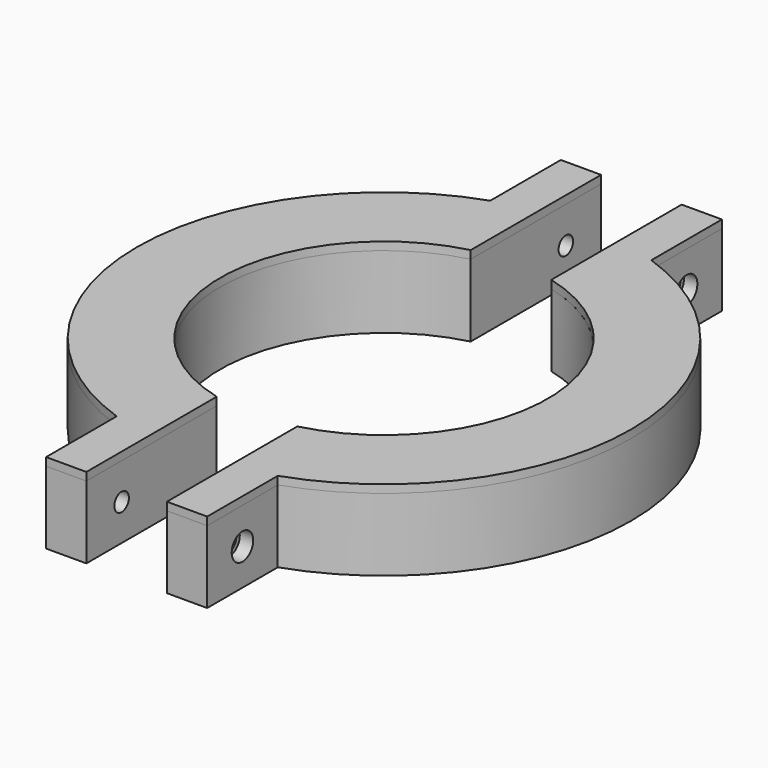
from build123d import *

# Parameters (mm, degrees)
F1_DEPTH      = 2
F2_DEPTH      = 25
F2_DEPTH_BACK = 2
F4_R          = 3.38
F5_DEPTH      = 122.001
F7_DEPTH      = 5
F9_DEPTH      = 3
F6_R          = 5
F6_R_2        = 3.38
F10_DEPTH     = 5


with BuildPart() as f1:
    # F0 (on Top) → F1 (new body)
    with BuildSketch(Plane.XY):
        with BuildLine():
            ThreePointArc((-30, -56.5331761004), (-64, 0), (-30, 56.5331761004))
            Line((-30, 56.5331761004), (-30, 83.7914076741))
            ThreePointArc((-30, 83.7914076741), (-89, 0), (-30, -83.7914076741))
            Line((-30, -83.7914076741), (-30, -56.5331761004))
        make_face()
    extrude(amount=-F1_DEPTH)

    # F0 (on Top) → F2 (join, two sides)
    with BuildSketch(Plane.XY) as f2_sk:
        with BuildLine():
            ThreePointArc((-30, -53.1130868996), (-61, 0), (-30, 53.1130868996))
            Line((-30, 53.1130868996), (-30, 56.5331761004))
            ThreePointArc((-30, 56.5331761004), (-64, 0), (-30, -56.5331761004))
            Line((-30, -56.5331761004), (-30, -53.1130868996))
        make_face()
        with BuildLine():
            ThreePointArc((-30, 53.1130868996), (-22.7000381841, 56.6189744383), (-15, 59.1269819964))
            Line((-15, 59.1269819964), (-15, 62.2173609212))
            ThreePointArc((-15, 62.2173609212), (-22.6787894137, 59.8470760416), (-30, 56.5331761004))
            Line((-30, 56.5331761004), (-30, 53.1130868996))
        make_face()
        with BuildLine():
            Line((-15, -87.7268487978), (-15, -62.2173609212))
            ThreePointArc((-15, -62.2173609212), (-22.6787894137, -59.8470760416), (-30, -56.5331761004))
            Line((-30, -56.5331761004), (-30, -83.7914076741))
            ThreePointArc((-30, -83.7914076741), (-22.5858788673, -86.0864569824), (-15, -87.7268487978))
        make_face()
        with BuildLine():
            Line((-15, -62.2173609212), (-15, -59.1269819964))
            ThreePointArc((-15, -59.1269819964), (-22.7000381841, -56.6189744383), (-30, -53.1130868996))
            Line((-30, -53.1130868996), (-30, -56.5331761004))
            ThreePointArc((-30, -56.5331761004), (-22.6787894137, -59.8470760416), (-15, -62.2173609212))
        make_face()
        with BuildLine():
            Line((-15, -90.768937418), (-15, -87.7268487978))
            ThreePointArc((-15, -87.7268487978), (-22.5858788673, -86.0864569824), (-30, -83.7914076741))
            Line((-30, -83.7914076741), (-30, -86.9712596206))
            ThreePointArc((-30, -86.9712596206), (-22.5799820452, -89.1860101744), (-15, -90.768937418))
        make_face()
        with BuildLine():
            Line((-15, -119.826041162), (-15, -90.768937418))
            ThreePointArc((-15, -90.768937418), (-22.5799820452, -89.1860101744), (-30, -86.9712596206))
            Line((-30, -86.9712596206), (-30, -119.826041162))
            Line((-30, -119.826041162), (-15, -119.826041162))
        make_face()
        with BuildLine():
            ThreePointArc((-30, -83.7914076741), (-89, 0), (-30, 83.7914076741))
            Line((-30, 83.7914076741), (-30, 86.9712596206))
            ThreePointArc((-30, 86.9712596206), (-92, 0), (-30, -86.9712596206))
            Line((-30, -86.9712596206), (-30, -83.7914076741))
        make_face()
        with BuildLine():
            ThreePointArc((-30, 56.5331761004), (-22.6787894137, 59.8470760416), (-15, 62.2173609212))
            Line((-15, 62.2173609212), (-15, 87.7268487978))
            ThreePointArc((-15, 87.7268487978), (-22.5858788673, 86.0864569824), (-30, 83.7914076741))
            Line((-30, 83.7914076741), (-30, 56.5331761004))
        make_face()
        with BuildLine():
            ThreePointArc((-30, 83.7914076741), (-22.5858788673, 86.0864569824), (-15, 87.7268487978))
            Line((-15, 87.7268487978), (-15, 90.768937418))
            ThreePointArc((-15, 90.768937418), (-22.5799820452, 89.1860101744), (-30, 86.9712596206))
            Line((-30, 86.9712596206), (-30, 83.7914076741))
        make_face()
        with BuildLine():
            ThreePointArc((-30, 86.9712596206), (-22.5799820452, 89.1860101744), (-15, 90.768937418))
            Line((-15, 90.768937418), (-15, 119.826041162))
            Line((-15, 119.826041162), (-30, 119.826041162))
            Line((-30, 119.826041162), (-30, 86.9712596206))
        make_face()
    extrude(amount=F2_DEPTH)
    extrude(f2_sk.sketch, amount=-F2_DEPTH_BACK)


with BuildPart() as f1b:
    # F0 (on Top) → F1, piece 2 (new body)
    with BuildSketch(Plane.XY):
        with BuildLine():
            Line((30, 83.7914076741), (30, 56.5331761004))
            ThreePointArc((30, 56.5331761004), (54.8452368032, 32.9848450049), (64, 0))
            ThreePointArc((64, 0), (54.8452368032, -32.9848450049), (30, -56.5331761004))
            Line((30, -56.5331761004), (30, -83.7914076741))
            ThreePointArc((30, -83.7914076741), (72.7701862029, -51.2396330978), (89, 0))
            ThreePointArc((89, 0), (72.7701862029, 51.2396330978), (30, 83.7914076741))
        make_face()
    extrude(amount=-F1_DEPTH)

    # F0 (on Top) → F2, piece 2 (join, two sides)
    with BuildSketch(Plane.XY) as f2_2_sk:
        with BuildLine():
            ThreePointArc((15, 59.1269819964), (22.7000381841, 56.6189744383), (30, 53.1130868996))
            Line((30, 53.1130868996), (30, 56.5331761004))
            ThreePointArc((30, 56.5331761004), (22.6787894137, 59.8470760416), (15, 62.2173609212))
            Line((15, 62.2173609212), (15, 59.1269819964))
        make_face()
        with BuildLine():
            ThreePointArc((30, 53.1130868996), (52.6830143405, 30.748983723), (61, 0))
            ThreePointArc((61, 0), (52.6830143405, -30.748983723), (30, -53.1130868996))
            Line((30, -53.1130868996), (30, -56.5331761004))
            ThreePointArc((30, -56.5331761004), (54.8452368032, -32.9848450049), (64, 0))
            ThreePointArc((64, 0), (54.8452368032, 32.9848450049), (30, 56.5331761004))
            Line((30, 56.5331761004), (30, 53.1130868996))
        make_face()
        with BuildLine():
            Line((30, -83.7914076741), (30, -56.5331761004))
            ThreePointArc((30, -56.5331761004), (22.6787894137, -59.8470760416), (15, -62.2173609212))
            Line((15, -62.2173609212), (15, -87.7268487978))
            ThreePointArc((15, -87.7268487978), (22.5858788673, -86.0864569824), (30, -83.7914076741))
        make_face()
        with BuildLine():
            Line((30, -56.5331761004), (30, -53.1130868996))
            ThreePointArc((30, -53.1130868996), (22.7000381841, -56.6189744383), (15, -59.1269819964))
            Line((15, -59.1269819964), (15, -62.2173609212))
            ThreePointArc((15, -62.2173609212), (22.6787894137, -59.8470760416), (30, -56.5331761004))
        make_face()
        with BuildLine():
            Line((30, -86.9712596206), (30, -83.7914076741))
            ThreePointArc((30, -83.7914076741), (22.5858788673, -86.0864569824), (15, -87.7268487978))
            Line((15, -87.7268487978), (15, -90.768937418))
            ThreePointArc((15, -90.768937418), (22.5799820452, -89.1860101744), (30, -86.9712596206))
        make_face()
        with BuildLine():
            Line((30, 86.9712596206), (30, 83.7914076741))
            ThreePointArc((30, 83.7914076741), (72.7701862029, 51.2396330978), (89, 0))
            ThreePointArc((89, 0), (72.7701862029, -51.2396330978), (30, -83.7914076741))
            Line((30, -83.7914076741), (30, -86.9712596206))
            ThreePointArc((30, -86.9712596206), (74.9132832013, -53.4041196913), (92, 0))
            ThreePointArc((92, 0), (74.9132832013, 53.4041196913), (30, 86.9712596206))
        make_face()
        with BuildLine():
            Line((30, -119.826041162), (30, -86.9712596206))
            ThreePointArc((30, -86.9712596206), (22.5799820452, -89.1860101744), (15, -90.768937418))
            Line((15, -90.768937418), (15, -119.826041162))
            Line((15, -119.826041162), (30, -119.826041162))
        make_face()
        with BuildLine():
            ThreePointArc((15, 62.2173609212), (22.6787894137, 59.8470760416), (30, 56.5331761004))
            Line((30, 56.5331761004), (30, 83.7914076741))
            ThreePointArc((30, 83.7914076741), (22.5858788673, 86.0864569824), (15, 87.7268487978))
            Line((15, 87.7268487978), (15, 62.2173609212))
        make_face()
        with BuildLine():
            ThreePointArc((15, 90.768937418), (22.5799820452, 89.1860101744), (30, 86.9712596206))
            Line((30, 86.9712596206), (30, 119.826041162))
            Line((30, 119.826041162), (15, 119.826041162))
            Line((15, 119.826041162), (15, 90.768937418))
        make_face()
        with BuildLine():
            ThreePointArc((15, 87.7268487978), (22.5858788673, 86.0864569824), (30, 83.7914076741))
            Line((30, 83.7914076741), (30, 86.9712596206))
            ThreePointArc((30, 86.9712596206), (22.5799820452, 89.1860101744), (15, 90.768937418))
            Line((15, 90.768937418), (15, 87.7268487978))
        make_face()
    extrude(amount=F2_DEPTH)
    extrude(f2_2_sk.sketch, amount=-F2_DEPTH_BACK)


with BuildPart() as f5_tool:
    # F4 (on face) → F5 (new body, through all)
    with BuildSketch(Plane(origin=(-30, 0, 0), x_dir=(0, -1, 0), z_dir=(-1, 0, 0))):
        with Locations((-103.3986503913, 11.5)):
            Circle(F4_R)
        with Locations((103.3986503913, 11.5)):
            Circle(F4_R)
    extrude(amount=-F5_DEPTH)


with BuildPart() as f1_1:
    add(f1.part)

    # F5: cut by f5_tool
    add(f5_tool.part, mode=Mode.SUBTRACT)

    # F4 (on face) → F7 (cut)
    with BuildSketch(Plane(origin=(-30, 0, 0), x_dir=(0, -1, 0), z_dir=(-1, 0, 0))):
        Polygon((-96.701868562, 11.4197101238), (-99.9807264042, 17.2594382497), (-106.6775082335, 17.3397281259), (-110.0954322206, 11.5802898762), (-106.8165743784, 5.7405617503), (-100.1197925491, 5.6602718741), align=None)
        with Locations((-103.3986503913, 11.5)):
            Circle(F4_R, mode=Mode.SUBTRACT)
        Polygon((106.6775082335, 17.3397281259), (99.9807264042, 17.2594382497), (96.701868562, 11.4197101238), (100.1197925491, 5.6602718741), (106.8165743784, 5.7405617503), (110.0954322206, 11.5802898762), align=None)
        with Locations((103.3986503913, 11.5)):
            Circle(F4_R, mode=Mode.SUBTRACT)
    extrude(amount=-F7_DEPTH, mode=Mode.SUBTRACT)


with BuildPart() as f1b_1:
    add(f1b.part)

    # F5: cut by f5_tool
    add(f5_tool.part, mode=Mode.SUBTRACT)

    # F6 (on face) → F10 (cut)
    with BuildSketch(Plane.YZ.offset(30)):
        with Locations((-103.3986503913, 11.5)):
            Circle(F6_R)
        with Locations((-103.3986503913, 11.5)):
            Circle(F6_R_2, mode=Mode.SUBTRACT)
        with Locations((103.3986503913, 11.5)):
            Circle(F6_R)
    extrude(amount=-F10_DEPTH, mode=Mode.SUBTRACT)


with BuildPart() as f9:
    # F8 (on face) → F9 (new body)
    with BuildSketch(Plane.XY.offset(25)):
        with BuildLine():
            Line((-15, 59.1269819964), (-15, 119.826041162))
            Line((-15, 119.826041162), (-30, 119.826041162))
            Line((-30, 119.826041162), (-30, 86.9712596206))
            ThreePointArc((-30, 86.9712596206), (-92, 0), (-30, -86.9712596206))
            Line((-30, -86.9712596206), (-30, -119.826041162))
            Line((-30, -119.826041162), (-15, -119.826041162))
            Line((-15, -119.826041162), (-15, -59.1269819964))
            ThreePointArc((-15, -59.1269819964), (-61, 0), (-15, 59.1269819964))
        make_face()
        with BuildLine():
            Line((-30, -56.5331761004), (-30, -83.7914076741))
            ThreePointArc((-30, -83.7914076741), (-89, 0), (-30, 83.7914076741))
            Line((-30, 83.7914076741), (-30, 56.5331761004))
            ThreePointArc((-30, 56.5331761004), (-64, 0), (-30, -56.5331761004))
        make_face(mode=Mode.SUBTRACT)
        with BuildLine():
            ThreePointArc((-30, 83.7914076741), (-89, 0), (-30, -83.7914076741))
            Line((-30, -83.7914076741), (-30, -56.5331761004))
            ThreePointArc((-30, -56.5331761004), (-64, 0), (-30, 56.5331761004))
            Line((-30, 56.5331761004), (-30, 83.7914076741))
        make_face()
    extrude(amount=F9_DEPTH)


with BuildPart() as f9b:
    # F8 (on face) → F9, piece 2 (new body)
    with BuildSketch(Plane.XY.offset(25)):
        with BuildLine():
            Line((30, 86.9712596206), (30, 119.826041162))
            Line((30, 119.826041162), (15, 119.826041162))
            Line((15, 119.826041162), (15, 59.1269819964))
            ThreePointArc((15, 59.1269819964), (61, 0), (15, -59.1269819964))
            Line((15, -59.1269819964), (15, -119.826041162))
            Line((15, -119.826041162), (30, -119.826041162))
            Line((30, -119.826041162), (30, -86.9712596206))
            ThreePointArc((30, -86.9712596206), (92, 0), (30, 86.9712596206))
        make_face()
    extrude(amount=F9_DEPTH)


solid = Compound([f1_1.part, f1b_1.part, f9.part, f9b.part])
